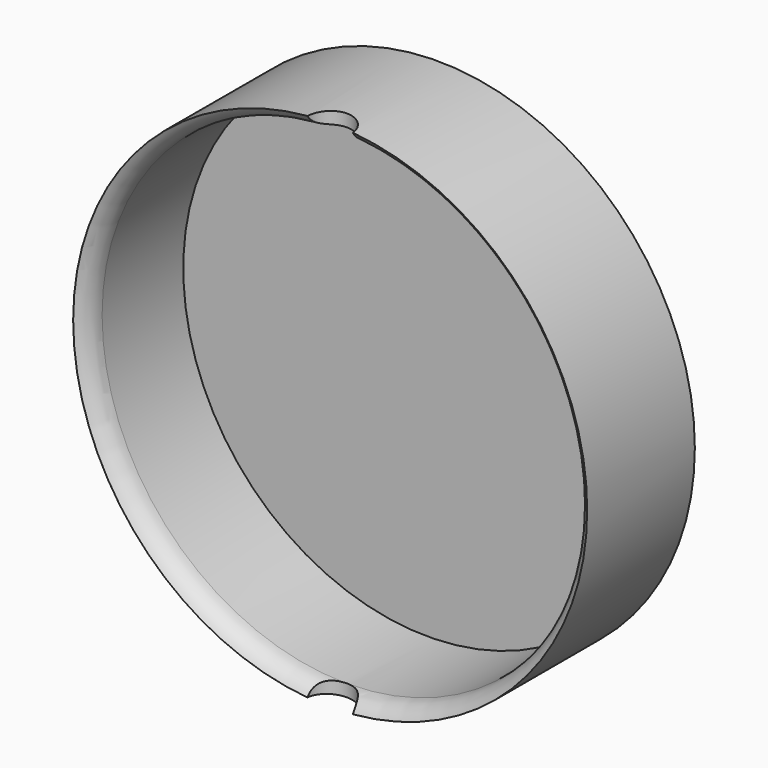
from build123d import *

# Parameters (mm, degrees)
F0_R          = 53.3590641314
F1_DEPTH      = 2.54
F2_R          = 53.3590641314
F2_R_2        = 50.8190641314
F3_DEPTH      = 25.4
F5_R          = 4.731473746
F6_DEPTH      = 53.3600641314
F6_DEPTH_BACK = 53.3600641314


# Not quite as in the source:
# - a fillet or chamfer that OpenCascade refuses, or shapes differently, is made with other operations: its cross-section is extruded or revolved along the edge and cut away or added


with BuildPart() as f1:
    # F0 (on Front) → F1 (new body)
    with BuildSketch(Plane.XZ):
        Circle(F0_R)
    extrude(amount=F1_DEPTH)

    # F2 (on face) → F3 (join)
    with BuildSketch(Plane.XZ.offset(2.54)):
        Circle(F2_R)
        Circle(F2_R_2, mode=Mode.SUBTRACT)
    extrude(amount=F3_DEPTH)

    # F4: fillet of radius 5.08 on 1 edges, made by hand

    # F4_s1 → F4_t2 (revolve, cut)
    with BuildSketch(Plane.XY):
        with BuildLine():
            ThreePointArc((53.3588640934, -27.9403463882), (51.4992986538, -26.0804748362), (50.8186641314, -23.5400334454))
            Line((50.8186641314, -23.5400334454), (50.3105275628, -23.5400334454))
            ThreePointArc((50.3105275628, -23.5400334454), (50.3109275628, -25.7400167227), (50.3109275628, -27.94))
            Line((50.3109275628, -27.94), (50.8190641314, -28.4481365685))
            ThreePointArc((50.8190641314, -28.4481365685), (52.0889641124, -28.4481365685), (53.104747521, -28.3803776825))
            Line((53.104747521, -28.3803776825), (53.3588640934, -27.9403463882))
        make_face()
    revolve(axis=Axis((0, -27.94, 0), (0, -1, 0)), mode=Mode.SUBTRACT)

    # F5 (on Top) → F6 (cut, two sides)
    with BuildSketch(Plane.XY) as f6_sk:
        with Locations((0, -28.3043142408)):
            Circle(F5_R)
    extrude(amount=-F6_DEPTH, mode=Mode.SUBTRACT)
    extrude(f6_sk.sketch, amount=F6_DEPTH_BACK, mode=Mode.SUBTRACT)


solid = f1.part
